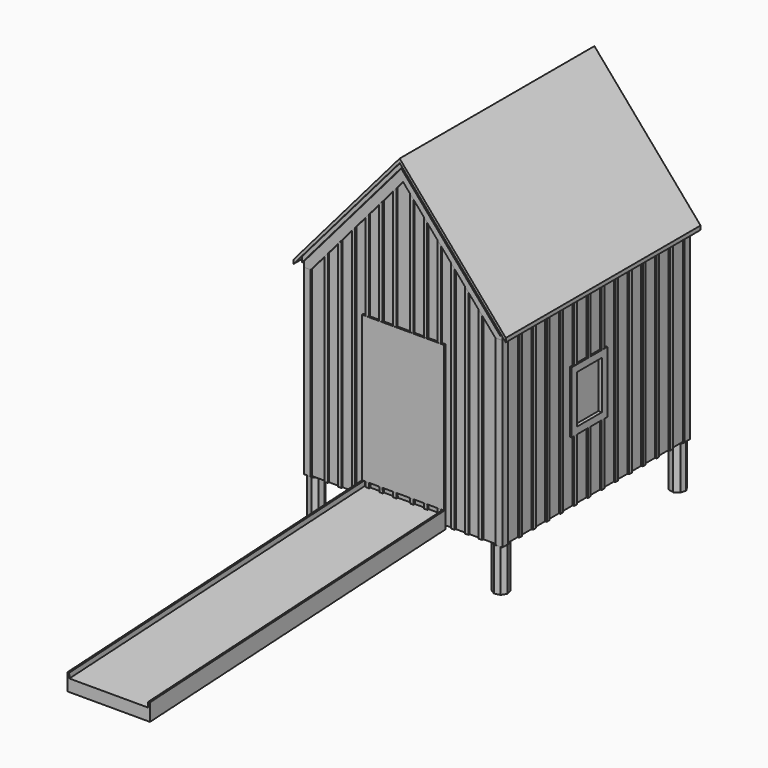
from build123d import *

# Parameters (mm, degrees)
F1_DEPTH    = 3606.8
F3_DEPTH    = 3606.801
F5_DEPTH    = 25.4
F7_DEPTH    = 25.4
F9_DEPTH    = 38.1
F11_DEPTH   = 38.1
F13_DEPTH   = 25.4
F15_DEPTH   = 25.4
F16_W       = 101.6
F16_H       = 101.6
F17_DEPTH   = 2701.3347888875
F18_W       = 22.86
F18_H       = 50.8
F19_DEPTH   = 2701.3347888875
F20_W       = 50.8
F20_H       = 22.86
F23_W       = 50.8
F23_H       = 2159
F23_W_2     = 152.4
F23_W_3     = 203.2
F24_DEPTH   = 25.4
F27_DEPTH   = 609.6
F27_FACE1_W = 1219.2
F27_FACE1_H = 254.3485758835
F29_DEPTH   = 76.2
F31_DEPTH   = 635
F32_W       = 660.4
F32_H       = 914.4
F33_DEPTH   = 25.4
F34_W       = 660.4
F34_H       = 914.4
F35_DEPTH   = 25.4
F36_W       = 457.2
F36_H       = 711.2
F37_DEPTH   = 50.8
F38_W       = 457.2
F38_H       = 711.2
F39_DEPTH   = 50.8
F40_W       = 812.8
F40_H       = 914.4
F41_DEPTH   = 25.4
F42_W       = 609.6
F42_H       = 711.2
F43_DEPTH   = 50.8


# Not quite as in the source:
# - a pattern or mirror of a feature is missing from the dataset's text; its kind, count and spacing are read off the source's solid


with BuildPart() as f1:
    # F0 (on Front) → F1 (new body)
    with BuildSketch(Plane.XZ):
        Polygon((0, 2794), (0, 0), (3144.52, 0), (3144.52, 2794), (1572.26, 4622.8), align=None)
    extrude(amount=-F1_DEPTH)

    # F2 (on face) → F3 (cut, through all)
    with BuildSketch(Plane.XZ):
        Polygon((101.6, 2701.3347888875), (101.6, 2853.7347888875), (0, 2735.5570829101), (0, 0), (127, 0), (127, 2701.3347888875), align=None)
        Polygon((3017.52, 2701.3347888875), (3017.52, 0), (3144.52, 0), (3144.52, 2735.5570829101), (3042.92, 2853.7347888875), (3042.92, 2701.3347888875), align=None)
    extrude(amount=-F3_DEPTH, mode=Mode.SUBTRACT)

    # F4 (on face) → F5 (cut)
    with BuildSketch(Plane.XZ):
        Polygon((1572.26, 4564.3570829101), (101.6, 2853.7347888875), (101.6, 2701.3347888875), (127, 2701.3347888875), (127, 0), (3017.52, 0), (3017.52, 2701.3347888875), (3042.92, 2701.3347888875), (3042.92, 2853.7347888875), align=None)
    extrude(amount=-F5_DEPTH, mode=Mode.SUBTRACT)

    # F6 (on face) → F7 (cut)
    with BuildSketch(Plane(origin=(0, 3606.8, 0), x_dir=(-1, 0, 0), z_dir=(0, 1, 0))):
        Polygon((-101.6, 2853.7347888875), (-1572.26, 4564.3570829101), (-3042.92, 2853.7347888875), (-3042.92, 2701.3347888875), (-3017.52, 2701.3347888875), (-3017.52, 0), (-127, 0), (-127, 2701.3347888875), (-101.6, 2701.3347888875), align=None)
    extrude(amount=-F7_DEPTH, mode=Mode.SUBTRACT)

    # F8 (on face) → F9 (cut)
    with BuildSketch(Plane.XZ.offset(-25.4)):
        Polygon((1572.26, 4486.4331934568), (101.6, 2775.8108994342), (101.6, 2701.3347888875), (127, 2701.3347888875), (127, 0), (3017.52, 0), (3017.52, 2701.3347888875), (3042.92, 2701.3347888875), (3042.92, 2775.8108994342), align=None)
    extrude(amount=-F9_DEPTH, mode=Mode.SUBTRACT)

    # F10 (on face) → F11 (cut)
    with BuildSketch(Plane(origin=(0, 3581.4, 0), x_dir=(-1, 0, 0), z_dir=(0, 1, 0))):
        Polygon((-101.6, 2775.8108994342), (-1572.26, 4486.4331934568), (-3042.92, 2775.8108994342), (-3042.92, 2701.3347888875), (-3017.52, 2701.3347888875), (-3017.52, 0), (-127, 0), (-127, 2701.3347888875), (-101.6, 2701.3347888875), align=None)
    extrude(amount=-F11_DEPTH, mode=Mode.SUBTRACT)

    # F12 (on face) → F13 (cut)
    with BuildSketch(Plane.XZ.offset(-63.5)):
        Polygon((205.0534812506, 2701.3347888875), (127, 2701.3347888875), (127, 0), (3017.52, 0), (3017.52, 2701.3347888875), (2939.4665187494, 2701.3347888875), (1572.26, 4291.6234698238), align=None)
    extrude(amount=-F13_DEPTH, mode=Mode.SUBTRACT)

    # F14 (on face) → F15 (cut)
    with BuildSketch(Plane(origin=(0, 3543.3, 0), x_dir=(-1, 0, 0), z_dir=(0, 1, 0))):
        Polygon((-127, 2701.3347888875), (-205.0534812506, 2701.3347888875), (-1572.26, 4291.6234698238), (-2939.4665187494, 2701.3347888875), (-3017.52, 2701.3347888875), (-3017.52, 0), (-127, 0), align=None)
    extrude(amount=-F15_DEPTH, mode=Mode.SUBTRACT)

    # F16 (on face) → F17 (join, through all)
    with BuildSketch(Plane(origin=(0, 0, 0), x_dir=(1, 0, 0), z_dir=(0, 0, -1))):
        with Locations((149.86, -116.84)):
            Rectangle(F16_W, F16_H)
        with Locations((149.86, -3489.96)):
            Rectangle(F16_W, F16_H)
        with Locations((2989.58, -3489.96)):
            Rectangle(F16_W, F16_H)
        with Locations((2989.58, -116.84)):
            Rectangle(F16_W, F16_H)
    extrude(amount=-F17_DEPTH)

    # F18 (on face) → F19 (join, through all)
    with BuildSketch(Plane(origin=(0, 0, 0), x_dir=(1, 0, 0), z_dir=(0, 0, -1))):
        with Locations((115.57, -3200.4)):
            Rectangle(F18_W, F18_H)
        with Locations((115.57, -2946.4)):
            Rectangle(F18_W, F18_H)
        with Locations((115.57, -2692.4)):
            Rectangle(F18_W, F18_H)
        with Locations((115.57, -2438.4)):
            Rectangle(F18_W, F18_H)
        with Locations((115.57, -2184.4)):
            Rectangle(F18_W, F18_H)
        with Locations((115.57, -1930.4)):
            Rectangle(F18_W, F18_H)
        with Locations((115.57, -1676.4)):
            Rectangle(F18_W, F18_H)
        with Locations((115.57, -1422.4)):
            Rectangle(F18_W, F18_H)
        with Locations((115.57, -1168.4)):
            Rectangle(F18_W, F18_H)
        with Locations((115.57, -914.4)):
            Rectangle(F18_W, F18_H)
        with Locations((115.57, -660.4)):
            Rectangle(F18_W, F18_H)
        with Locations((115.57, -406.4)):
            Rectangle(F18_W, F18_H)
        with Locations((3028.95, -3200.4)):
            Rectangle(F18_W, F18_H)
        with Locations((3028.95, -2946.4)):
            Rectangle(F18_W, F18_H)
        with Locations((3028.95, -2692.4)):
            Rectangle(F18_W, F18_H)
        with Locations((3028.95, -2438.4)):
            Rectangle(F18_W, F18_H)
        with Locations((3028.95, -2184.4)):
            Rectangle(F18_W, F18_H)
        with Locations((3028.95, -1930.4)):
            Rectangle(F18_W, F18_H)
        with Locations((3028.95, -1676.4)):
            Rectangle(F18_W, F18_H)
        with Locations((3028.95, -1422.4)):
            Rectangle(F18_W, F18_H)
        with Locations((3028.95, -1168.4)):
            Rectangle(F18_W, F18_H)
        with Locations((3028.95, -914.4)):
            Rectangle(F18_W, F18_H)
        with Locations((3028.95, -660.4)):
            Rectangle(F18_W, F18_H)
        with Locations((3028.95, -406.4)):
            Rectangle(F18_W, F18_H)
    extrude(amount=-F19_DEPTH)

    # F20 (on face) → F21 (join, up to the next surface of F1)
    with BuildSketch(Plane(origin=(0, 0, 0), x_dir=(1, 0, 0), z_dir=(0, 0, -1))):
        with Locations((429.26, -77.47)):
            Rectangle(F20_W, F20_H)
        with Locations((632.46, -77.47)):
            Rectangle(F20_W, F20_H)
        with Locations((835.66, -77.47)):
            Rectangle(F20_W, F20_H)
        with Locations((1038.86, -77.47)):
            Rectangle(F20_W, F20_H)
        with Locations((1242.06, -77.47)):
            Rectangle(F20_W, F20_H)
        with Locations((1445.26, -77.47)):
            Rectangle(F20_W, F20_H)
        with Locations((632.46, -3529.33)):
            Rectangle(F20_W, F20_H)
        with Locations((429.26, -3529.33)):
            Rectangle(F20_W, F20_H)
        with Locations((1445.26, -3529.33)):
            Rectangle(F20_W, F20_H)
        with Locations((835.66, -3529.33)):
            Rectangle(F20_W, F20_H)
        with Locations((1242.06, -3529.33)):
            Rectangle(F20_W, F20_H)
        with Locations((1038.86, -3529.33)):
            Rectangle(F20_W, F20_H)
    f21 = extrude(until=Until.NEXT, dir=(0, 0, 1))

    # F21_copies: F21 across plane
    add(f21.mirror(Plane(origin=(1572.26, 0, 0), x_dir=(0, 0, 1), z_dir=(1, 0, 0))))

    # F23 (on face) → F24 (join)
    with BuildSketch(Plane.XZ.offset(-88.9)):
        with Locations((988.06, 1282.7)):
            Rectangle(F23_W, F23_H)
        with Locations((1038.86, 1282.7)):
            Rectangle(F23_W, F23_H)
        with Locations((1140.46, 1282.7)):
            Rectangle(F23_W_2, F23_H)
        with Locations((1242.06, 1282.7)):
            Rectangle(F23_W, F23_H)
        with Locations((1343.66, 1282.7)):
            Rectangle(F23_W_2, F23_H)
        with Locations((1445.26, 1282.7)):
            Rectangle(F23_W, F23_H)
        with Locations((1572.26, 1282.7)):
            Rectangle(F23_W_3, F23_H)
        with Locations((1699.26, 1282.7)):
            Rectangle(F23_W, F23_H)
        with Locations((1800.86, 1282.7)):
            Rectangle(F23_W_2, F23_H)
        with Locations((1902.46, 1282.7)):
            Rectangle(F23_W, F23_H)
        with Locations((2004.06, 1282.7)):
            Rectangle(F23_W_2, F23_H)
        with Locations((2105.66, 1282.7)):
            Rectangle(F23_W, F23_H)
        with Locations((2156.46, 1282.7)):
            Rectangle(F23_W, F23_H)
    extrude(amount=F24_DEPTH)

    # F26 (on plane+point) → F27 (join, symmetric)
    with BuildSketch(Plane(origin=(1572.26, 0, 0), x_dir=(0, -1, 0), z_dir=(-1, 0, 0))):
        Polygon((5389.9810794775, -83.9359903313), (-88.9, 203.2), (-88.9, -51.1485758835), (5389.9810794775, -338.2845662148), align=None)
    extrude(amount=F27_DEPTH, both=True)

    # F28 (on face) + F27_face1 (on face) → F29 (cut)
    with BuildSketch(Plane(origin=(0, -10.3765901171, 197.9971343772), x_dir=(1, 0, 0), z_dir=(0, -0.0523359562, 0.9986295348))):
        Polygon((1013.46, 99.4128319482), (988.06, 99.4128319482), (988.06, -5386.9871680518), (2156.46, -5386.9871680518), (2156.46, 99.4128319482), (2131.06, 99.4128319482), (2131.06, 76.5214601187), (2080.26, 76.5214601187), (2080.26, 99.4128319482), (1927.86, 99.4128319482), (1927.86, 76.5214601187), (1877.06, 76.5214601187), (1877.06, 99.4128319482), (1724.66, 99.4128319482), (1724.66, 76.5214601187), (1673.86, 76.5214601187), (1673.86, 99.4128319482), (1470.66, 99.4128319482), (1470.66, 76.5214601187), (1419.86, 76.5214601187), (1419.86, 99.4128319482), (1267.46, 99.4128319482), (1267.46, 76.5214601187), (1216.66, 76.5214601187), (1216.66, 99.4128319482), (1064.26, 99.4128319482), (1064.26, 76.5214601187), (1013.46, 76.5214601187), align=None)
    with BuildSketch(Plane(origin=(1572.26, -5389.9810794775, -211.110278273), x_dir=(1, 0, 0), z_dir=(0, -1, 0))):
        Rectangle(F27_FACE1_W, F27_FACE1_H)
    extrude(amount=-F29_DEPTH, dir=(0, -0.0523359562, 0.9986295348), mode=Mode.SUBTRACT)

    # F30 (on face) → F31 (join)
    with BuildSketch(Plane(origin=(0, 0, 0), x_dir=(1, 0, 0), z_dir=(0, 0, -1))):
        Polygon((267.6723175869, -254.1895704566), (311.7846523674, -182.5070264384), (292.2895704566, -100.6276824131), (220.6070264384, -56.5153476326), (138.7276824131, -76.0104295434), (94.6153476326, -147.6929735616), (114.1104295434, -229.5723175869), (185.7929735616, -273.6846523674), align=None)
        Polygon((2876.8476824131, -254.1895704566), (2958.7270264383, -273.6846523674), (3030.4095704566, -229.5723175869), (3049.9046523674, -147.6929735616), (3005.7923175869, -76.0104295434), (2923.9129735616, -56.5153476326), (2852.2304295434, -100.6276824131), (2832.7353476326, -182.5070264384), align=None)
        Polygon((267.6723175869, -3352.6104295434), (185.7929735616, -3333.1153476326), (114.1104295434, -3377.2276824131), (94.6153476326, -3459.1070264384), (138.7276824131, -3530.7895704566), (220.6070264384, -3550.2846523674), (292.2895704566, -3506.1723175869), (311.7846523674, -3424.2929735616), align=None)
        Polygon((2876.8476824131, -3352.6104295434), (2832.7353476326, -3424.2929735616), (2852.2304295434, -3506.1723175869), (2923.9129735616, -3550.2846523674), (3005.7923175869, -3530.7895704566), (3049.9046523674, -3459.1070264384), (3030.4095704566, -3377.2276824131), (2958.7270264383, -3333.1153476326), align=None)
    extrude(amount=F31_DEPTH)

    # F32 (on face) → F33 (join)
    with BuildSketch(Plane(origin=(127, 0, 0), x_dir=(0, -1, 0), z_dir=(-1, 0, 0))):
        with Locations((-1676.4, 1371.6)):
            Rectangle(F32_W, F32_H)
    extrude(amount=F33_DEPTH)

    # F34 (on face) → F35 (join)
    with BuildSketch(Plane.YZ.offset(3017.52)):
        with Locations((1676.4, 1371.6)):
            Rectangle(F34_W, F34_H)
    extrude(amount=F35_DEPTH)

    # F36 (on face) → F37 (cut)
    with BuildSketch(Plane.YZ.offset(3042.92)):
        with Locations((1676.4, 1371.6)):
            Rectangle(F36_W, F36_H)
    extrude(amount=-F37_DEPTH, mode=Mode.SUBTRACT)

    # F38 (on face) → F39 (cut)
    with BuildSketch(Plane(origin=(101.6, 0, 0), x_dir=(0, -1, 0), z_dir=(-1, 0, 0))):
        with Locations((-1676.4, 1371.6)):
            Rectangle(F38_W, F38_H)
    extrude(amount=-F39_DEPTH, mode=Mode.SUBTRACT)

    # F40 (on face) → F41 (join)
    with BuildSketch(Plane(origin=(0, 3517.9, 0), x_dir=(-1, 0, 0), z_dir=(0, 1, 0))):
        with Locations((-1572.26, 1371.6)):
            Rectangle(F40_W, F40_H)
    extrude(amount=F41_DEPTH)

    # F42 (on face) → F43 (cut)
    with BuildSketch(Plane(origin=(0, 3543.3, 0), x_dir=(-1, 0, 0), z_dir=(0, 1, 0))):
        with Locations((-1572.26, 1371.6)):
            Rectangle(F42_W, F42_H)
    extrude(amount=-F43_DEPTH, mode=Mode.SUBTRACT)


solid = f1.part
